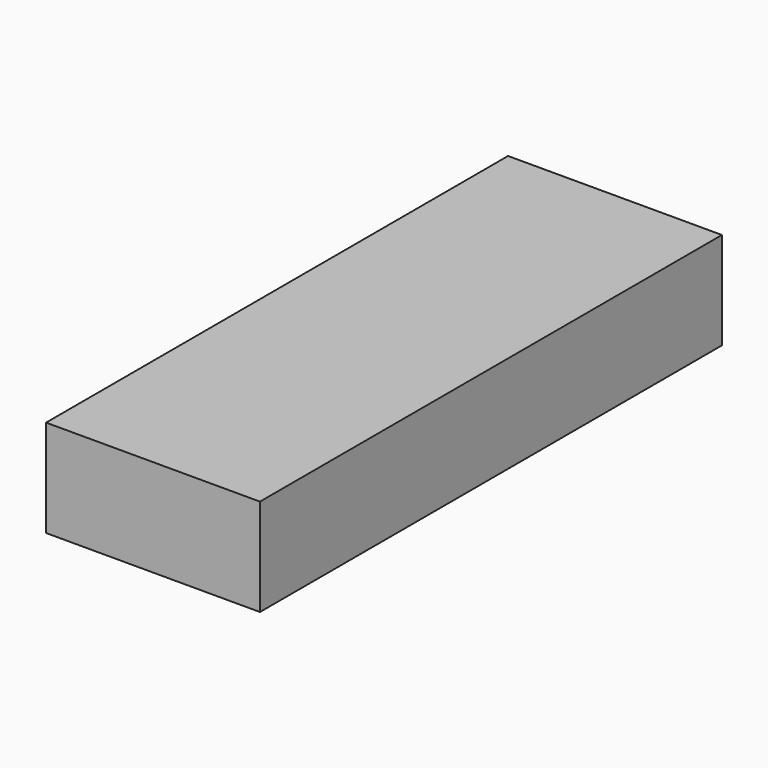
from build123d import *

# Parameters (mm, degrees)
F2_W     = 22
F2_H     = 6.4
F2_H_2   = 12.3
F2_H_3   = 22
F4_DEPTH = 5


with BuildPart() as f4:
    # F2 (on Top) → F4 (new body, symmetric)
    with BuildSketch(Plane.XY):
        with Locations((0, 26.5)):
            Rectangle(F2_W, F2_H)
        with Locations((0, 17.15)):
            Rectangle(F2_W, F2_H_2)
        Rectangle(F2_W, F2_H_3)
        Polygon((-11, -25.98033873), (-11, -29.7), (11, -29.7), (11, -23.3), (-11, -23.3), align=None)
        with Locations((0, -17.15)):
            Rectangle(F2_W, F2_H_2)
    extrude(amount=F4_DEPTH, both=True)


solid = f4.part
